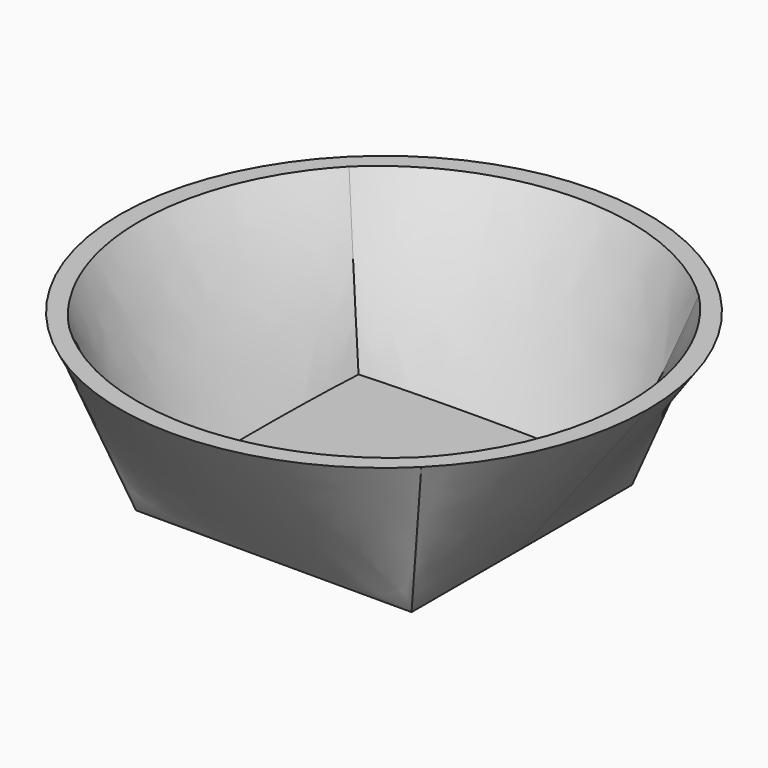
from build123d import *

# Parameters (mm, degrees)
F2_R = 43.0981164558
F1_W = 45
F1_H = 45
F4_T = 2.5


# Not quite as in the source:
# - a shell that OpenCascade refuses in one call is made with other operations: the cavity is built on its own and cut out


with BuildPart() as f3:
    # F2 (on offset) → F3 section 0
    with BuildSketch(Plane.XY.offset(26.7)):
        Circle(F2_R)
    # F1 (on Top) → F3 section 1
    with BuildSketch(Plane.XY):
        Rectangle(F1_W, F1_H)
    loft()

    # F4: shell of thickness 2.5, made by hand


with BuildPart() as f4_core1:
    # F4_t2: copy of F3
    add(f3.part)

    # the walls: a layer under each face that stays
    f4_faces = [f4_core1.faces().sort_by_distance(p)[0] for p in [
        (31.1587338374, 13.8714675651, 13.35),
        (0, 32.7990582263, 13.35),
        (-32.7990582263, 0, 13.35),
        (0, -32.7990582263, 13.35),
        (31.1587338374, -13.8714675651, 13.35),
        (0, 0, 0),
    ]]
    thicken(f4_faces, amount=-F4_T, mode=Mode.SUBTRACT)


with BuildPart() as f3_1:
    add(f3.part)

    # what is left inside the walls is the cavity
    f4_cavity = [f4_core1.part.solids().sort_by_distance(p)[0] for p in [
        (0, -13.313542, 26.675),
    ]]
    add(f4_cavity, mode=Mode.SUBTRACT)


solid = f3_1.part
